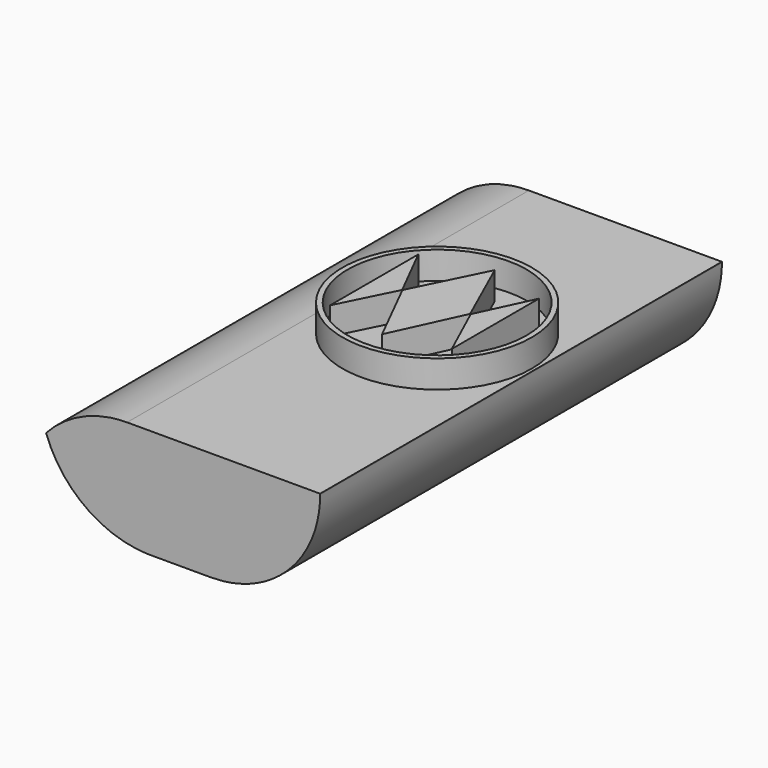
from build123d import *

# Parameters (mm, degrees)
F0_W        = 62.0055571198
F0_H        = 91.1606
F2_W        = 43.9132880419
F2_H        = 91.28
F4_R        = 20
F5_R        = 20
F6_T1_DEPTH = 247.1570875446
F8_R        = 17.2017157063
F8_R_2      = 16.2487468326
F9_DEPTH    = 5
F10_DEPTH   = 5


# Not quite as in the source:
# - a fillet or chamfer that OpenCascade refuses, or shapes differently, is made with other operations: its cross-section is extruded or revolved along the edge and cut away or added


with BuildPart() as f3:
    # F0 (on Top) → F3 section 0
    with BuildSketch(Plane.XY):
        with Locations((3.4252367914, -5.9738955829)):
            Rectangle(F0_W, F0_H)
    # F2 (on offset) → F3 section 1
    with BuildSketch(Plane.XY.offset(20)):
        with Locations((12.6207480207, -6.1396389759)):
            Rectangle(F2_W, F2_H)
    loft()

    # F4
    f4_edges = [f3.edges().sort_by_distance(p)[0] for p in [
        (-9.335896, -6.139639, 20),
    ]]
    fillet(f4_edges, radius=F4_R)

    # F5
    f5_edges = [f3.edges().sort_by_distance(p)[0] for p in [
        (34.428015, -5.973896, 0),
    ]]
    fillet(f5_edges, radius=F5_R)

    # F6: fillet of radius 20 on 1 edges, made by hand

    # F6_s2 → F6_t1 (cut)
    with BuildSketch(Plane.XZ.offset(-117.6046481894)):
        with BuildLine():
            ThreePointArc((3.6217557404, 0), (-7.9875678865, 3.7143128813), (-15.2848254843, 13.4776395073))
            Line((-15.2848254843, 13.4776395073), (-27.5775417686, 0))
            Line((-27.5775417686, 0), (3.6217557404, 0))
        make_face()
    extrude(amount=F6_T1_DEPTH, mode=Mode.SUBTRACT)

    # F8 (on offset) → F9 (join)
    with BuildSketch(Plane.XY.offset(20)):
        with Locations((16.8321914971, -3.0107519124)):
            Circle(F8_R)
        with Locations((16.8321914971, -3.0107519124)):
            Circle(F8_R_2, mode=Mode.SUBTRACT)
        Polygon((5.5154971778, 6.8484889343), (5.5154971778, -13.2129238918), (10.5462484062, -3.106220687), align=None)
        Polygon((27.3772925138, -12.8699932247), (27.3772925138, 6.9342213683), (22.7957628667, -2.8306879103), align=None)
    extrude(amount=F9_DEPTH)

    # F8 (on offset) → F10 (join)
    with BuildSketch(Plane.XY.offset(20)):
        Polygon((17.0036572963, 9.8491283134), (10.6022227556, -3.106220687), (16.8321914971, -15.5277010053), (22.6763673127, -2.8306879103), align=None)
    extrude(amount=F10_DEPTH)


solid = f3.part
